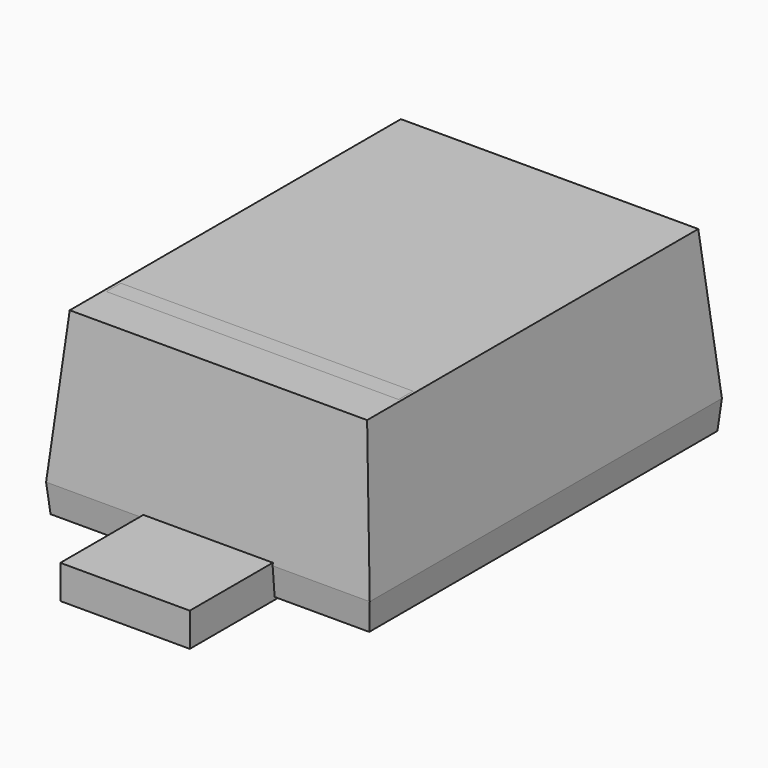
from build123d import *

# Parameters (mm, degrees)
F0_W          = 0.5
F0_H          = 0.55
F1_DEPTH      = 0.13
F0_W_2        = 0.35
F3_W          = 1.25
F3_H          = 1.7
F4_DEPTH      = 0.58
F4_DEPTH_BACK = 0.11
F5_SIZE2      = 0.58
F5_SIZE       = 0.0507434248
F6_SIZE2      = 0.10999
F6_SIZE       = 0.009614
F7_W          = 1.1285131503
F7_H          = 0.07
F8_DEPTH      = 0.01


# Not quite as in the source:
# - a fillet or chamfer is up to 0.001 mm smaller than in the source, because OpenCascade refuses the exact size


with BuildPart() as f1:
    # F0 (on Top) → F1 (new body)
    with BuildSketch(Plane.XY):
        with Locations((0, -0.975)):
            Rectangle(F0_W, F0_H)
    extrude(amount=F1_DEPTH)


with BuildPart() as f1b:
    # F0 (on Top) → F1, piece 2 (new body)
    with BuildSketch(Plane.XY):
        with Locations((0, 0.975)):
            Rectangle(F0_W_2, F0_H)
    extrude(amount=F1_DEPTH)


with BuildPart() as f4:
    # F3 (on offset) → F4 (new body, two sides)
    with BuildSketch(Plane.XY.offset(0.12)) as f4_sk:
        Rectangle(F3_W, F3_H)
    extrude(amount=F4_DEPTH)
    extrude(f4_sk.sketch, amount=-F4_DEPTH_BACK)

    # F5
    f5_edges = [f4.edges().sort_by_distance(p)[0] for p in [
        (0, -0.85, 0.7),
        (0.625, 0, 0.7),
        (0, 0.85, 0.7),
        (-0.625, 0, 0.7),
    ]]
    f5_side = f4.faces().sort_by_distance((0, 0, 0.7))[0]
    chamfer(f5_edges, length=F5_SIZE, length2=F5_SIZE2, reference=f5_side)

    # F6 (size 0.009623753 and 0.11 in the source; OpenCascade refuses exactly that, so slightly less here)
    f6_edges = [f4.edges().sort_by_distance(p)[0] for p in [
        (0.625, 0, 0.01),
        (0, 0.85, 0.01),
        (-0.625, 0, 0.01),
        (0, -0.85, 0.01),
    ]]
    f6_side = f4.faces().sort_by_distance((0, 0, 0.01))[0]
    chamfer(f6_edges, length=F6_SIZE, length2=F6_SIZE2, reference=f6_side)


with BuildPart() as f8:
    # F7 (on face) → F8 (new body)
    with BuildSketch(Plane.XY.offset(0.7)):
        with Locations((0, -0.6)):
            Rectangle(F7_W, F7_H)
    extrude(amount=-F8_DEPTH)


with BuildPart() as f4_1:
    add(f4.part)

    # F9: cut F8
    add(f8.part, mode=Mode.SUBTRACT)


solid = Compound([f1.part, f1b.part, f8.part, f4_1.part])
